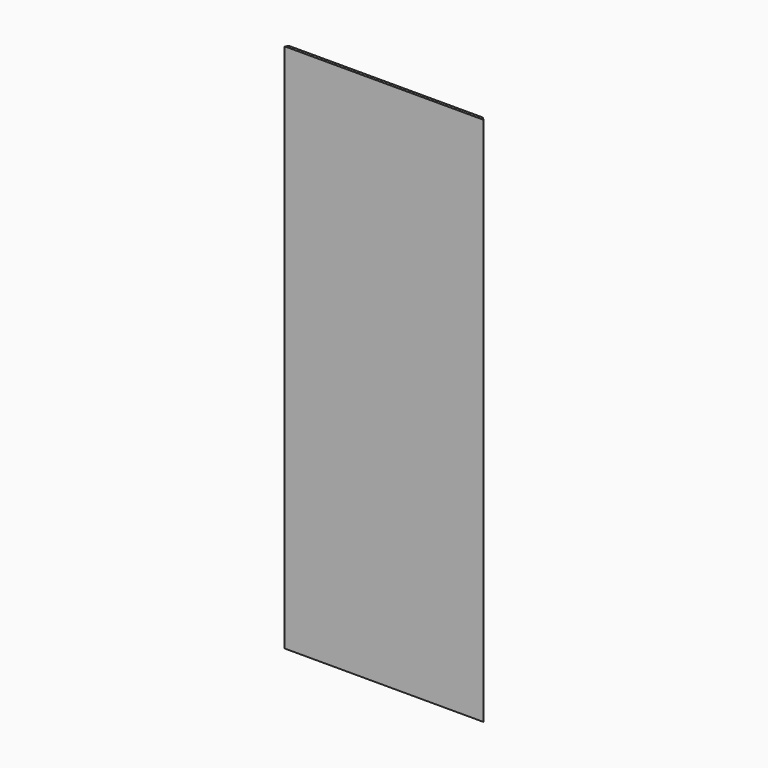
from build123d import *

# Parameters (mm, degrees)
F0_W     = 457.2
F0_H     = 1219.2
F1_DEPTH = 6.35
F2_SIZE  = 6.34999
F3_SIZE  = 6.34999


# Not quite as in the source:
# - a fillet or chamfer is up to 0.001 mm smaller than in the source, because OpenCascade refuses the exact size


with BuildPart() as f1:
    # F0 (on Front) → F1 (new body)
    with BuildSketch(Plane.XZ):
        Rectangle(F0_W, F0_H)
    extrude(amount=F1_DEPTH)

    # F2 (size 6.35 in the source; OpenCascade refuses exactly that, so slightly less here)
    f2_edges = [f1.edges().sort_by_distance(p)[0] for p in [
        (-228.6, 0, 0),
    ]]
    chamfer(f2_edges, length=F2_SIZE)

    # F3 (size 6.35 in the source; OpenCascade refuses exactly that, so slightly less here)
    f3_edges = [f1.edges().sort_by_distance(p)[0] for p in [
        (228.6, 0, 0),
    ]]
    chamfer(f3_edges, length=F3_SIZE)


solid = f1.part
